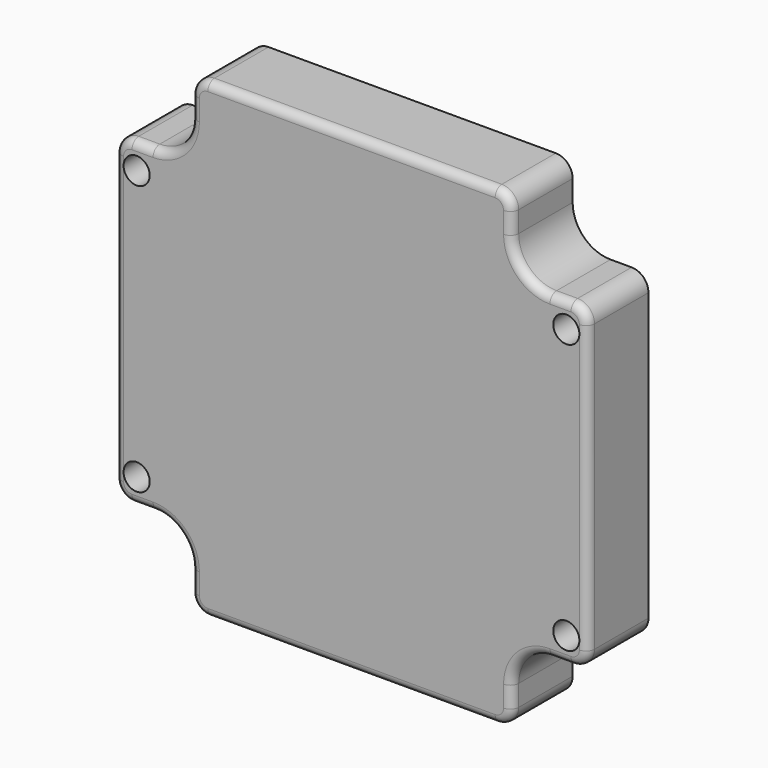
from build123d import *

# Parameters (mm, degrees)
F0_R     = 1.55
F1_DEPTH = 9
F2_R     = 0.99999


# Not quite as in the source:
# - a fillet or chamfer is up to 0.001 mm smaller than in the source, because OpenCascade refuses the exact size


with BuildPart() as f1:
    # F0 (on Front) → F1 (new body)
    with BuildSketch(Plane.XZ):
        with BuildLine():
            Line((17.05, 28), (-17.05, 28))
            ThreePointArc((-17.05, 28), (-18.4642135624, 27.4142135624), (-19.05, 26))
            Line((-19.05, 26), (-19.05, 23.5))
            ThreePointArc((-19.05, 23.5), (-20.3680194847, 20.3180194847), (-23.55, 19))
            Line((-23.55, 19), (-26.05, 19))
            ThreePointArc((-26.05, 19), (-27.4642135624, 18.4142135624), (-28.05, 17))
            Line((-28.05, 17), (-28.05, -17))
            ThreePointArc((-28.05, -17), (-27.4642135624, -18.4142135624), (-26.05, -19))
            Line((-26.05, -19), (-23.55, -19))
            ThreePointArc((-23.55, -19), (-20.3680194847, -20.3180194847), (-19.05, -23.5))
            Line((-19.05, -23.5), (-19.05, -26))
            ThreePointArc((-19.05, -26), (-18.4642135624, -27.4142135624), (-17.05, -28))
            Line((-17.05, -28), (17.05, -28))
            ThreePointArc((17.05, -28), (18.4642135624, -27.4142135624), (19.05, -26))
            Line((19.05, -26), (19.05, -23.5))
            ThreePointArc((19.05, -23.5), (20.3680194847, -20.3180194847), (23.55, -19))
            Line((23.55, -19), (26.05, -19))
            ThreePointArc((26.05, -19), (27.4642135624, -18.4142135624), (28.05, -17))
            Line((28.05, -17), (28.05, 17))
            ThreePointArc((28.05, 17), (27.4642135624, 18.4142135624), (26.05, 19))
            Line((26.05, 19), (23.55, 19))
            ThreePointArc((23.55, 19), (20.3680194847, 20.3180194847), (19.05, 23.5))
            Line((19.05, 23.5), (19.05, 26))
            ThreePointArc((19.05, 26), (18.4642135624, 27.4142135624), (17.05, 28))
        make_face()
        with Locations((-25.5, -16)):
            Circle(F0_R, mode=Mode.SUBTRACT)
        with Locations((25.5, -16)):
            Circle(F0_R, mode=Mode.SUBTRACT)
        with Locations((-25.5, 16)):
            Circle(F0_R, mode=Mode.SUBTRACT)
        with Locations((25.5, 16)):
            Circle(F0_R, mode=Mode.SUBTRACT)
    extrude(amount=F1_DEPTH)

    # F2 (radius 1 in the source; OpenCascade refuses exactly that, so slightly less here)
    f2_edges = [f1.edges().sort_by_distance(p)[0] for p in [
        (-27.464214, -9, 18.414214),
    ]]
    fillet(f2_edges, radius=F2_R)


solid = f1.part
